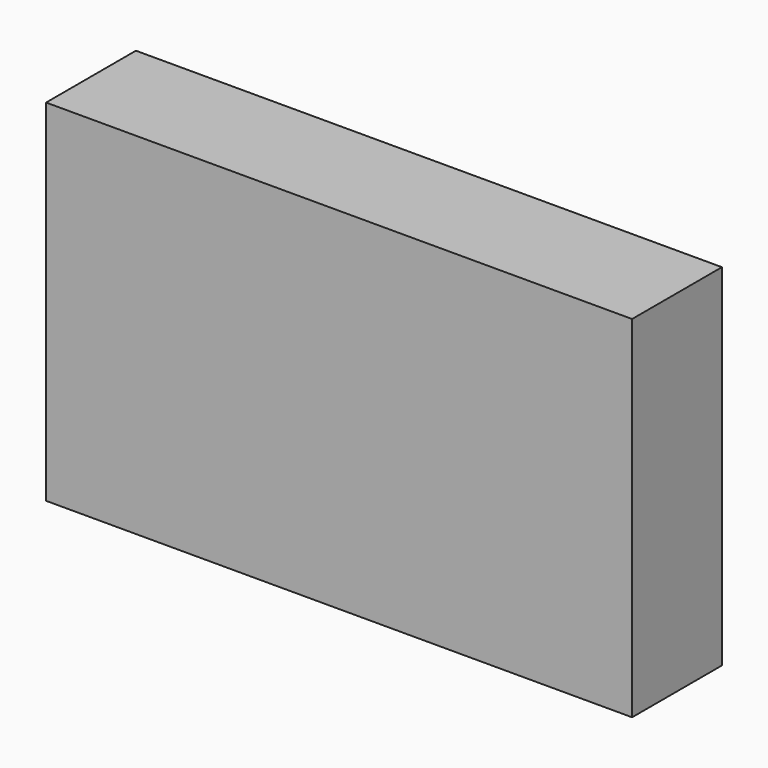
from build123d import *

# Parameters (mm, degrees)
F0_W     = 130.488038063
F0_H     = 78.0766904354
F1_DEPTH = 25
F3_D     = 12.7
F3_DEPTH = 12
F3_TIP   = 3.8154649308


# Not quite as in the source:
# - a length typed as a fraction of an inch, garbled in the dataset ("3 / 203.2 mm" for 3/8 in), is restored


with BuildPart() as f1:
    # F0 (on Front) → F1 (new body)
    with BuildSketch(Plane.XZ):
        with Locations((4.5927464962, -2.1641068161)):
            Rectangle(F0_W, F0_H)
    extrude(amount=F1_DEPTH)

    # F3
    with Locations(Plane(origin=(0, 0, 0), x_dir=(1, 0, 0), z_dir=(0, 1, 0))):
        with Locations((-13.1143694744, 18.479084596), (-5.4509616457, -20.7668524235), (49.2379032075, 5.5906269699)):
            Hole(F3_D / 2, depth=F3_DEPTH)
            with Locations((0, 0, -(F3_DEPTH + F3_TIP / 2))):  # 118° drill point
                Cone(0, F3_D / 2, F3_TIP, mode=Mode.SUBTRACT)


solid = f1.part
